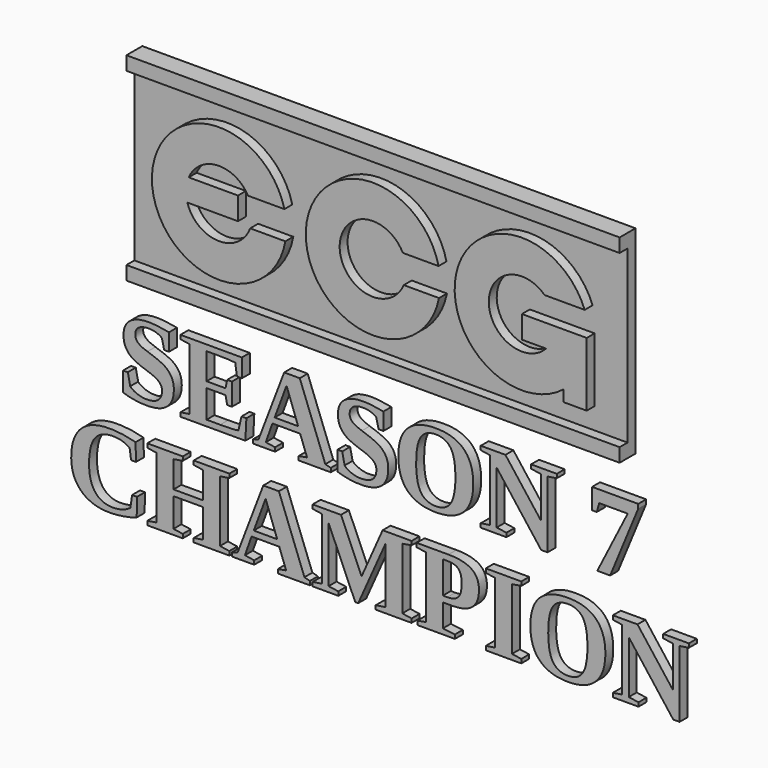
from build123d import *

# Parameters (mm, degrees)
F0_TEXT_SIZE = 11.1111111111
F0_W         = 49.7207662151
F0_H         = 1.3843632213
F0_H_2       = 17.2312735574
F1_DEPTH     = 1
F2_DEPTH     = 2


# Not quite as in the source:
# - Text() gives the source's letters only with a copy of the font that has no kerning and outlines rounded to 1/6400 em; it was checked with that copy


with BuildPart() as f1:
    # F0 (on Front) → F1 (new body)
    with BuildSketch(Plane.XZ):
        with Locations((-38.1412851537, -58.2452112551)):
            Text('SEASON 7', F0_TEXT_SIZE, font='Tinos', font_style=FontStyle.BOLD, text_align=(TextAlign.LEFT, TextAlign.BOTTOM))
        with Locations((-43.3235354722, -68.962700665)):
            Text('CHAMPION', F0_TEXT_SIZE, font='Tinos', font_style=FontStyle.BOLD, text_align=(TextAlign.LEFT, TextAlign.BOTTOM))
        with Locations((-11.552377495, -46.5704380042)):
            Rectangle(F0_W, F0_H)
        with Locations((-11.552377495, -37.2626196149)):
            Rectangle(F0_W, F0_H_2)
        with BuildLine():
            ThreePointArc((-20.3908795189, -38.5673468951), (-33.8406010497, -37.6249411484), (-20.4898783318, -35.7430961081))
            Line((-20.4898783318, -35.7430961081), (-24.1550842785, -35.7430961081))
            ThreePointArc((-24.1550842785, -35.7430961081), (-27.2418171577, -34.0487583484), (-30.1336247029, -36.0577753799))
            Line((-30.1336247029, -36.0577753799), (-25.16651678, -36.0577753799))
            Line((-25.16651678, -36.0577753799), (-25.16651678, -38.3372576581))
            Line((-25.16651678, -38.3372576581), (-30.2716747131, -38.3372576581))
            ThreePointArc((-30.2716747131, -38.3372576581), (-27.1874582706, -40.7286057921), (-23.9378587658, -38.5673468951))
            Line((-23.9378587658, -38.5673468951), (-20.3908795189, -38.5673468951))
        make_face(mode=Mode.SUBTRACT)
        with BuildLine():
            ThreePointArc((-4.9004491104, -38.5673468951), (-18.3301652426, -37.3724274422), (-4.9462051675, -35.7430961081))
            Line((-4.9462051675, -35.7430961081), (-8.5494970928, -35.7430961081))
            ThreePointArc((-8.5494970928, -35.7430961081), (-14.9157448064, -37.3809527305), (-8.450131676, -38.5673468951))
            Line((-8.450131676, -38.5673468951), (-4.9004491104, -38.5673468951))
        make_face(mode=Mode.SUBTRACT)
        with BuildLine():
            ThreePointArc((7.6327018584, -42.6011109922), (-3.0773806533, -35.4517246536), (9.7851025932, -34.8384407391))
            Line((9.7851025932, -34.8384407391), (5.7484859002, -34.8384407391))
            ThreePointArc((5.7484859002, -34.8384407391), (0.1189099625, -37.3660237386), (5.8937906105, -39.5412374199))
            Line((5.8937906105, -39.5412374199), (3.4548410849, -39.5412374199))
            Line((3.4548410849, -39.5412374199), (3.4548410849, -37.2629517714))
            Line((3.4548410849, -37.2629517714), (6.7923641612, -37.2629517714))
            Line((6.7923641612, -37.2629517714), (9.9891936574, -37.2629517714))
            Line((9.9891936574, -37.2629517714), (9.9891936574, -43.7193689139))
            Line((9.9891936574, -43.7193689139), (7.6327018584, -43.7193689139))
            Line((7.6327018584, -43.7193689139), (7.6327018584, -42.6011109922))
        make_face(mode=Mode.SUBTRACT)
        with BuildLine():
            Line((-24.1550842785, -35.7430961081), (-20.4898783318, -35.7430961081))
            ThreePointArc((-20.4898783318, -35.7430961081), (-33.8406010497, -37.6249411484), (-20.3908795189, -38.5673468951))
            Line((-20.3908795189, -38.5673468951), (-23.9378587658, -38.5673468951))
            ThreePointArc((-23.9378587658, -38.5673468951), (-27.1874582706, -40.7286057921), (-30.2716747131, -38.3372576581))
            Line((-30.2716747131, -38.3372576581), (-25.16651678, -38.3372576581))
            Line((-25.16651678, -38.3372576581), (-25.16651678, -36.0577753799))
            Line((-25.16651678, -36.0577753799), (-30.1336247029, -36.0577753799))
            ThreePointArc((-30.1336247029, -36.0577753799), (-27.2418171577, -34.0487583484), (-24.1550842785, -35.7430961081))
        make_face()
        with BuildLine():
            Line((-8.5494970928, -35.7430961081), (-4.9462051675, -35.7430961081))
            ThreePointArc((-4.9462051675, -35.7430961081), (-18.3301652426, -37.3724274422), (-4.9004491104, -38.5673468951))
            Line((-4.9004491104, -38.5673468951), (-8.450131676, -38.5673468951))
            ThreePointArc((-8.450131676, -38.5673468951), (-14.9157448064, -37.3809527305), (-8.5494970928, -35.7430961081))
        make_face()
        with BuildLine():
            Line((5.7484859002, -34.8384407391), (9.7851025932, -34.8384407391))
            ThreePointArc((9.7851025932, -34.8384407391), (-3.0773806533, -35.4517246536), (7.6327018584, -42.6011109922))
            Line((7.6327018584, -42.6011109922), (7.6327018584, -43.7193689139))
            Line((7.6327018584, -43.7193689139), (9.9891936574, -43.7193689139))
            Line((9.9891936574, -43.7193689139), (9.9891936574, -37.2629517714))
            Line((9.9891936574, -37.2629517714), (6.7923641612, -37.2629517714))
            Line((6.7923641612, -37.2629517714), (3.4548410849, -37.2629517714))
            Line((3.4548410849, -37.2629517714), (3.4548410849, -39.5412374199))
            Line((3.4548410849, -39.5412374199), (5.8937906105, -39.5412374199))
            ThreePointArc((5.8937906105, -39.5412374199), (0.1189099625, -37.3660237386), (5.7484859002, -34.8384407391))
        make_face()
        with Locations((-11.552377495, -27.9548012255)):
            Rectangle(F0_W, F0_H)
    extrude(amount=F1_DEPTH)

    # F0 (on Front) → F2 (join)
    with BuildSketch(Plane.XZ):
        with Locations((-11.552377495, -46.5704380042)):
            Rectangle(F0_W, F0_H)
        with Locations((-11.552377495, -27.9548012255)):
            Rectangle(F0_W, F0_H)
        with BuildLine():
            Line((5.7484859002, -34.8384407391), (9.7851025932, -34.8384407391))
            ThreePointArc((9.7851025932, -34.8384407391), (-3.0773806533, -35.4517246536), (7.6327018584, -42.6011109922))
            Line((7.6327018584, -42.6011109922), (7.6327018584, -43.7193689139))
            Line((7.6327018584, -43.7193689139), (9.9891936574, -43.7193689139))
            Line((9.9891936574, -43.7193689139), (9.9891936574, -37.2629517714))
            Line((9.9891936574, -37.2629517714), (6.7923641612, -37.2629517714))
            Line((6.7923641612, -37.2629517714), (3.4548410849, -37.2629517714))
            Line((3.4548410849, -37.2629517714), (3.4548410849, -39.5412374199))
            Line((3.4548410849, -39.5412374199), (5.8937906105, -39.5412374199))
            ThreePointArc((5.8937906105, -39.5412374199), (0.1189099625, -37.3660237386), (5.7484859002, -34.8384407391))
        make_face()
        with BuildLine():
            Line((-8.5494970928, -35.7430961081), (-4.9462051675, -35.7430961081))
            ThreePointArc((-4.9462051675, -35.7430961081), (-18.3301652426, -37.3724274422), (-4.9004491104, -38.5673468951))
            Line((-4.9004491104, -38.5673468951), (-8.450131676, -38.5673468951))
            ThreePointArc((-8.450131676, -38.5673468951), (-14.9157448064, -37.3809527305), (-8.5494970928, -35.7430961081))
        make_face()
        with BuildLine():
            Line((-24.1550842785, -35.7430961081), (-20.4898783318, -35.7430961081))
            ThreePointArc((-20.4898783318, -35.7430961081), (-33.8406010497, -37.6249411484), (-20.3908795189, -38.5673468951))
            Line((-20.3908795189, -38.5673468951), (-23.9378587658, -38.5673468951))
            ThreePointArc((-23.9378587658, -38.5673468951), (-27.1874582706, -40.7286057921), (-30.2716747131, -38.3372576581))
            Line((-30.2716747131, -38.3372576581), (-25.16651678, -38.3372576581))
            Line((-25.16651678, -38.3372576581), (-25.16651678, -36.0577753799))
            Line((-25.16651678, -36.0577753799), (-30.1336247029, -36.0577753799))
            ThreePointArc((-30.1336247029, -36.0577753799), (-27.2418171577, -34.0487583484), (-24.1550842785, -35.7430961081))
        make_face()
    extrude(amount=F2_DEPTH)


solid = f1.part
